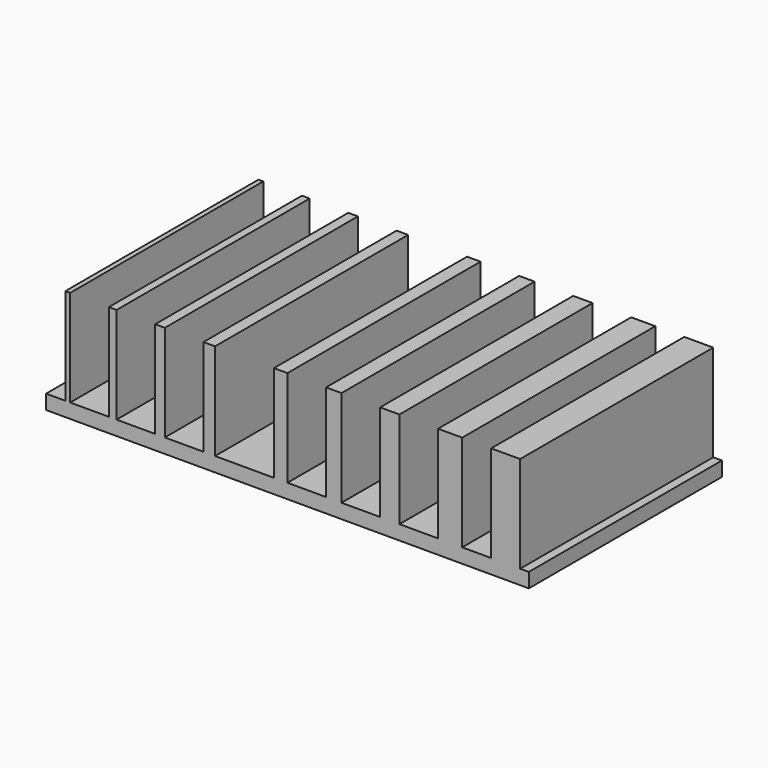
from build123d import *

# Parameters (mm, degrees)
F0_W     = 50
F0_H     = 1.5
F1_DEPTH = 25
F3_W     = 0.5
F3_H     = 25
F3_W_2   = 0.8
F3_W_3   = 1
F3_W_4   = 1.4
F3_W_5   = 1.2
F3_W_6   = 1.6
F3_W_7   = 2
F3_W_8   = 2.5
F3_W_9   = 3
F4_DEPTH = 10


with BuildPart() as f1:
    # F0 (on Front) → F1 (new body)
    with BuildSketch(Plane.XZ):
        with Locations((25, 0.75)):
            Rectangle(F0_W, F0_H)
    extrude(amount=-F1_DEPTH)

    # F3 (on offset) → F4 (join)
    with BuildSketch(Plane.XY.offset(1.5)):
        with Locations((2.25, 12.5)):
            Rectangle(F3_W, F3_H)
        with Locations((6.9, 12.5)):
            Rectangle(F3_W_2, F3_H)
        with Locations((11.8, 12.5)):
            Rectangle(F3_W_3, F3_H)
        with Locations((24.3, 12.5)):
            Rectangle(F3_W_4, F3_H)
        with Locations((16.9, 12.5)):
            Rectangle(F3_W_5, F3_H)
        with Locations((29.8, 12.5)):
            Rectangle(F3_W_6, F3_H)
        with Locations((35.6, 12.5)):
            Rectangle(F3_W_7, F3_H)
        with Locations((41.85, 12.5)):
            Rectangle(F3_W_8, F3_H)
        with Locations((47.6, 12.5)):
            Rectangle(F3_W_9, F3_H)
    extrude(amount=F4_DEPTH)


solid = f1.part
